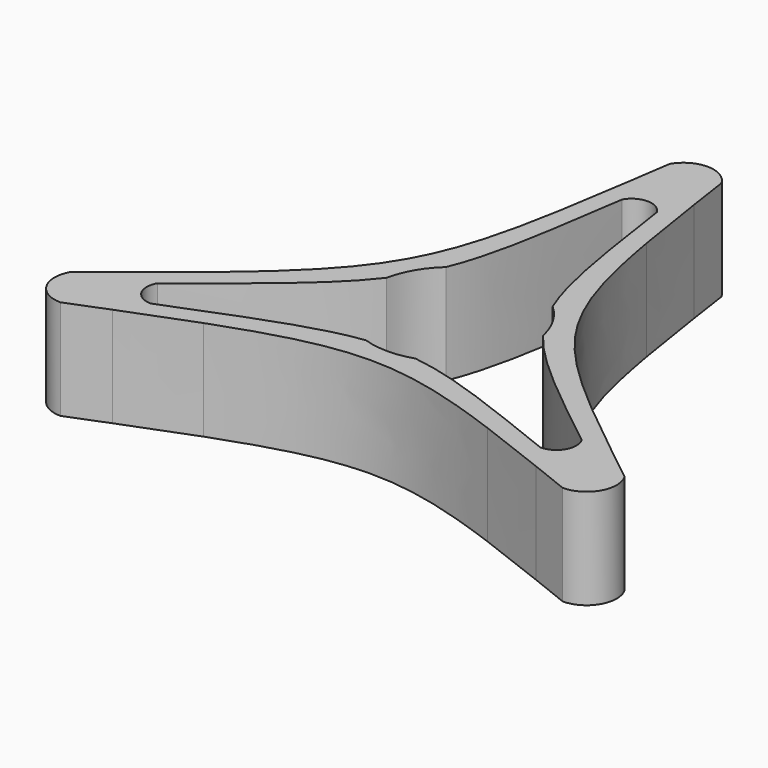
from build123d import *

# Parameters (mm, degrees)
F1_DEPTH = 10


# Not quite as in the source:
# - a feature of the source that left no trace in its solid (it failed there, or was rolled back) is left out


with BuildPart() as f1:
    # F0 (on Top) → F1 (new body)
    with BuildSketch(Plane.XY):
        with BuildLine():
            ThreePointArc((5.3398427629, 5.9570193274), (6.9282032303, 4), (7.8288514498, 1.6459298212))
            add(Edge.make_bspline(
                [(7.8288514498, 1.6459298212), (10.3819017266, -1.689149351), (14.3784307752, -4.8466401497), (21.2176223927, -10.25)],
                knots=[22.7730577605, 22.7730577605, 22.7730577605, 22.7730577605, 38.9711431703, 38.9711431703, 38.9711431703, 38.9711431703], degree=3))
            Line((21.2176223927, -10.25), (18.5700532559, -5.6642757385))
            add(Edge.make_bspline(
                [(18.5700532559, -5.6642757385), (8.8931150266, 2.4300062697), (6.5510046742, 6.486660397), (4.3796199444, 18.9142757385)],
                knots=[8.5821930458, 8.5821930458, 8.5821930458, 8.5821930458, 41.6472803737, 41.6472803737, 41.6472803737, 41.6472803737], degree=3))
            Line((4.3796199444, 18.9142757385), (1.7320508076, 23.5))
            add(Edge.make_bspline(
                [(1.7320508076, 23.5), (2.991901895, 14.8754063927), (3.7281046145, 9.8355653103), (5.3398427629, 5.9570193274)],
                knots=[0, 0, 0, 0, 16.1980854098, 16.1980854098, 16.1980854098, 16.1980854098], degree=3))
        make_face()
        with BuildLine():
            add(Edge.make_bspline(
                [(2.4890086869, -7.6029491486), (6.6537971121, -8.1464159593), (11.3865288802, -10.0287662431), (19.4855715851, -13.25)],
                knots=[22.7730577605, 22.7730577605, 22.7730577605, 22.7730577605, 38.9711431703, 38.9711431703, 38.9711431703, 38.9711431703], degree=3))
            ThreePointArc((2.4890086869, -7.6029491486), (0, -8), (-2.4890086869, -7.6029491486))
            add(Edge.make_bspline(
                [(-19.4855715852, -13.25), (-11.3865288802, -10.0287662431), (-6.6537971121, -8.1464159593), (-2.4890086869, -7.6029491486)],
                knots=[0, 0, 0, 0, 16.1980854098, 16.1980854098, 16.1980854098, 16.1980854098], degree=3))
            Line((-19.4855715852, -13.25), (-14.1904333115, -13.25))
            add(Edge.make_bspline(
                [(-14.1904333115, -13.25), (-2.3421103524, -8.9166666667), (2.3421103524, -8.9166666667), (14.1904333115, -13.25)],
                knots=[8.5821930458, 8.5821930458, 8.5821930458, 8.5821930458, 41.6472803737, 41.6472803737, 41.6472803737, 41.6472803737], degree=3))
            Line((14.1904333115, -13.25), (19.4855715851, -13.25))
        make_face()
        with BuildLine():
            Line((18.5700532559, -5.6642757385), (21.2176223927, -10.25))
            ThreePointArc((21.2176223927, -10.25), (21.2176223927, -12.25), (19.4855715851, -13.25))
            Line((19.4855715851, -13.25), (14.1904333115, -13.25))
            add(Edge.make_bspline(
                [(14.1904333115, -13.25), (16.2714670553, -14.0111045817), (18.573507913, -14.9058892059), (21.174191051, -15.9343538726)],
                knots=[41.6472803737, 41.6472803737, 41.6472803737, 41.6472803737, 47.4548164026, 47.4548164026, 47.4548164026, 47.4548164026], degree=3))
            ThreePointArc((21.174191051, -15.9343538726), (22.9496732003, -13.25), (24.386650772, -10.3702104184))
            add(Edge.make_bspline(
                [(24.386650772, -10.3702104184), (22.1956326748, -8.6321850871), (20.2697060304, -7.0859515359), (18.5700532559, -5.6642757385)],
                knots=[2.7746570169, 2.7746570169, 2.7746570169, 2.7746570169, 8.5821930458, 8.5821930458, 8.5821930458, 8.5821930458], degree=3))
        make_face()
        with BuildLine():
            ThreePointArc((-7.8288514498, 1.6459298212), (-6.9282032303, 4), (-5.3398427629, 5.9570193274))
            add(Edge.make_bspline(
                [(-1.7320508076, 23.5), (-2.991901895, 14.8754063927), (-3.7281046145, 9.8355653103), (-5.3398427629, 5.9570193274)],
                knots=[0, 0, 0, 0, 16.1980854098, 16.1980854098, 16.1980854098, 16.1980854098], degree=3))
            Line((-1.7320508076, 23.5), (-4.3796199444, 18.9142757385))
            add(Edge.make_bspline(
                [(-4.3796199444, 18.9142757385), (-6.5510046742, 6.486660397), (-8.8931150266, 2.4300062697), (-18.5700532559, -5.6642757385)],
                knots=[8.5821930458, 8.5821930458, 8.5821930458, 8.5821930458, 41.6472803737, 41.6472803737, 41.6472803737, 41.6472803737], degree=3))
            Line((-18.5700532559, -5.6642757385), (-21.2176223927, -10.25))
            add(Edge.make_bspline(
                [(-7.8288514498, 1.6459298212), (-10.3819017266, -1.689149351), (-14.3784307752, -4.8466401497), (-21.2176223927, -10.25)],
                knots=[22.7730577605, 22.7730577605, 22.7730577605, 22.7730577605, 38.9711431703, 38.9711431703, 38.9711431703, 38.9711431703], degree=3))
        make_face()
        with BuildLine():
            ThreePointArc((-1.7320508076, 23.5), (0, 24.5), (1.7320508076, 23.5))
            Line((1.7320508076, 23.5), (4.3796199444, 18.9142757385))
            add(Edge.make_bspline(
                [(4.3796199444, 18.9142757385), (3.9982389752, 21.0970561175), (3.6221247618, 23.5380742929), (3.2124597211, 26.304564291)],
                knots=[41.6472803737, 41.6472803737, 41.6472803737, 41.6472803737, 47.4548164026, 47.4548164026, 47.4548164026, 47.4548164026], degree=3))
            ThreePointArc((3.2124597211, 26.304564291), (0, 26.5), (-3.2124597211, 26.304564291))
            add(Edge.make_bspline(
                [(-3.2124597211, 26.304564291), (-3.6221247618, 23.5380742929), (-3.9982389752, 21.0970561175), (-4.3796199444, 18.9142757385)],
                knots=[2.7746570169, 2.7746570169, 2.7746570169, 2.7746570169, 8.5821930458, 8.5821930458, 8.5821930458, 8.5821930458], degree=3))
            Line((-4.3796199444, 18.9142757385), (-1.7320508076, 23.5))
        make_face()
        with BuildLine():
            Line((-14.1904333115, -13.25), (-19.4855715852, -13.25))
            ThreePointArc((-19.4855715852, -13.25), (-21.2176223927, -12.25), (-21.2176223927, -10.25))
            Line((-21.2176223927, -10.25), (-18.5700532559, -5.6642757385))
            add(Edge.make_bspline(
                [(-18.5700532559, -5.6642757385), (-20.2697060304, -7.0859515359), (-22.1956326748, -8.6321850871), (-24.386650772, -10.3702104184)],
                knots=[41.6472803737, 41.6472803737, 41.6472803737, 41.6472803737, 47.4548164026, 47.4548164026, 47.4548164026, 47.4548164026], degree=3))
            ThreePointArc((-24.386650772, -10.3702104184), (-22.9496732003, -13.25), (-21.174191051, -15.9343538726))
            add(Edge.make_bspline(
                [(-21.174191051, -15.9343538726), (-18.573507913, -14.9058892059), (-16.2714670553, -14.0111045817), (-14.1904333115, -13.25)],
                knots=[2.7746570169, 2.7746570169, 2.7746570169, 2.7746570169, 8.5821930458, 8.5821930458, 8.5821930458, 8.5821930458], degree=3))
        make_face()
        with BuildLine():
            add(Edge.make_bspline(
                [(27.7128129211, -13), (26.540759526, -12.0747363675), (25.433449915, -11.2005839464), (24.386650772, -10.3702104184)],
                knots=[0, 0, 0, 0, 2.7746570169, 2.7746570169, 2.7746570169, 2.7746570169], degree=3))
            ThreePointArc((24.386650772, -10.3702104184), (22.9496732003, -13.25), (21.174191051, -15.9343538726))
            add(Edge.make_bspline(
                [(21.174191051, -15.9343538726), (22.4167151923, -16.425721759), (23.7274082013, -16.9476038015), (25.1147367097, -17.5)],
                knots=[47.4548164026, 47.4548164026, 47.4548164026, 47.4548164026, 50.2294734195, 50.2294734195, 50.2294734195, 50.2294734195], degree=3))
            ThreePointArc((25.1147367097, -17.5), (27.7128129211, -16), (27.7128129211, -13))
        make_face()
        with BuildLine():
            ThreePointArc((-3.2124597211, 26.304564291), (0, 26.5), (3.2124597211, 26.304564291))
            add(Edge.make_bspline(
                [(3.2124597211, 26.304564291), (3.0167347227, 27.6263057055), (2.8133513247, 29.0223401691), (2.5980762114, 30.5)],
                knots=[47.4548164026, 47.4548164026, 47.4548164026, 47.4548164026, 50.2294734195, 50.2294734195, 50.2294734195, 50.2294734195], degree=3))
            ThreePointArc((2.5980762114, 30.5), (0, 32), (-2.5980762114, 30.5))
            add(Edge.make_bspline(
                [(-2.5980762114, 30.5), (-2.8133513247, 29.0223401691), (-3.0167347227, 27.6263057055), (-3.2124597211, 26.304564291)],
                knots=[0, 0, 0, 0, 2.7746570169, 2.7746570169, 2.7746570169, 2.7746570169], degree=3))
        make_face()
        with BuildLine():
            add(Edge.make_bspline(
                [(-25.1147367097, -17.5), (-23.7274082013, -16.9476038015), (-22.4167151923, -16.425721759), (-21.174191051, -15.9343538726)],
                knots=[0, 0, 0, 0, 2.7746570169, 2.7746570169, 2.7746570169, 2.7746570169], degree=3))
            ThreePointArc((-21.174191051, -15.9343538726), (-22.9496732003, -13.25), (-24.386650772, -10.3702104184))
            add(Edge.make_bspline(
                [(-24.386650772, -10.3702104184), (-25.433449915, -11.2005839464), (-26.540759526, -12.0747363675), (-27.7128129211, -13)],
                knots=[47.4548164026, 47.4548164026, 47.4548164026, 47.4548164026, 50.2294734195, 50.2294734195, 50.2294734195, 50.2294734195], degree=3))
            ThreePointArc((-27.7128129211, -13), (-27.7128129211, -16), (-25.1147367097, -17.5))
        make_face()
    extrude(amount=F1_DEPTH)


solid = f1.part
